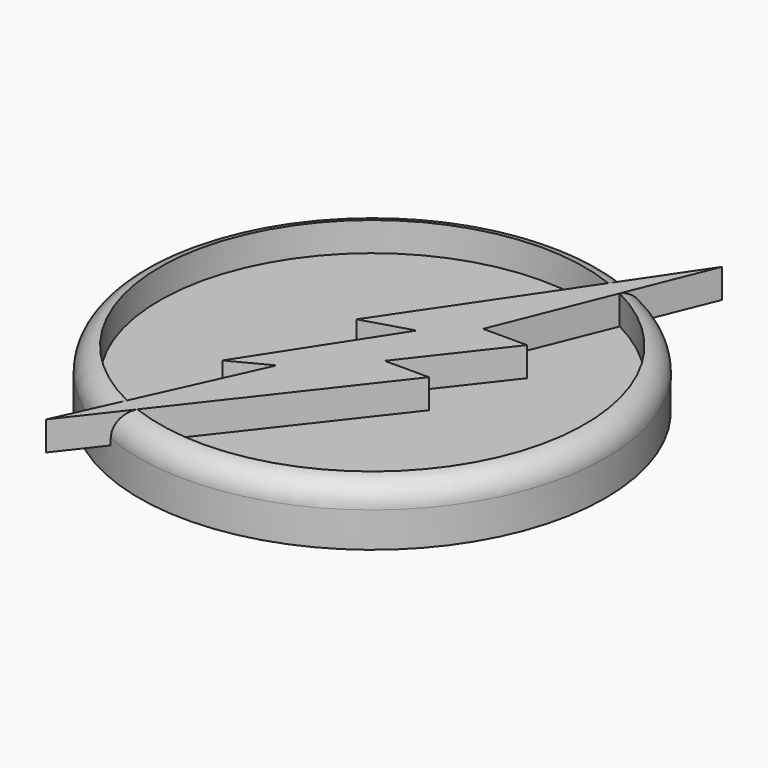
from build123d import *

# Parameters (mm, degrees)
F0_R     = 46.303997109
F1_DEPTH = 6.35
F0_R_2   = 50.7773250867
F2_DEPTH = 12.7
F5_DEPTH = 6.35


# Not quite as in the source:
# - a fillet or chamfer that OpenCascade refuses, or shapes differently, is made with other operations: its cross-section is extruded or revolved along the edge and cut away or added


with BuildPart() as f1:
    # F0 (on Top) → F1 (new body)
    with BuildSketch(Plane.XY):
        Circle(F0_R)
    extrude(amount=F1_DEPTH)

    # F0 (on Top) → F2 (join)
    with BuildSketch(Plane.XY):
        Circle(F0_R_2)
        Circle(F0_R, mode=Mode.SUBTRACT)
    extrude(amount=F2_DEPTH)

    # F3: fillet of radius 5.08 on 1 edges, made by hand

    # F3_s1 → F3_t2 (revolve, cut)
    with BuildSketch(Plane.XZ):
        with BuildLine():
            ThreePointArc((50.7773250867, 7.6563555778), (49.4978706971, 11.0271497073), (46.303997109, 12.7))
            Line((46.303997109, 12.7), (46.3161305494, 12.8008728884))
            ThreePointArc((46.3161305494, 12.8008728884), (48.5406610978, 12.8016), (50.7773250867, 12.8016))
            Line((50.7773250867, 12.8016), (50.8789250867, 12.7))
            Line((50.8789250867, 12.7), (50.8789250867, 7.6563555778))
            Line((50.8789250867, 7.6563555778), (50.7773250867, 7.6563555778))
        make_face()
    revolve(axis=Axis((0, 0, 12.7), (0, 0, 1)), mode=Mode.SUBTRACT)

    # F4 (on face) → F5 (join)
    with BuildSketch(Plane.XY.offset(6.35)):
        Polygon((-8.1779062748, -15.8028278183), (-26.3735784938, -55.8334334653), (14.7386826575, -3.0078946147), (5.1134219393, -3.0078946147), (20.4086864271, 16.6451374931), (10.8284205198, 16.6451374931), (28.2742083073, 59.8571076989), (-8.1779062748, 5.9409798123), (2.4016224779, 9.0941041708), (-16.5434218943, -20.15289478), align=None)
    extrude(amount=F5_DEPTH)


solid = f1.part
